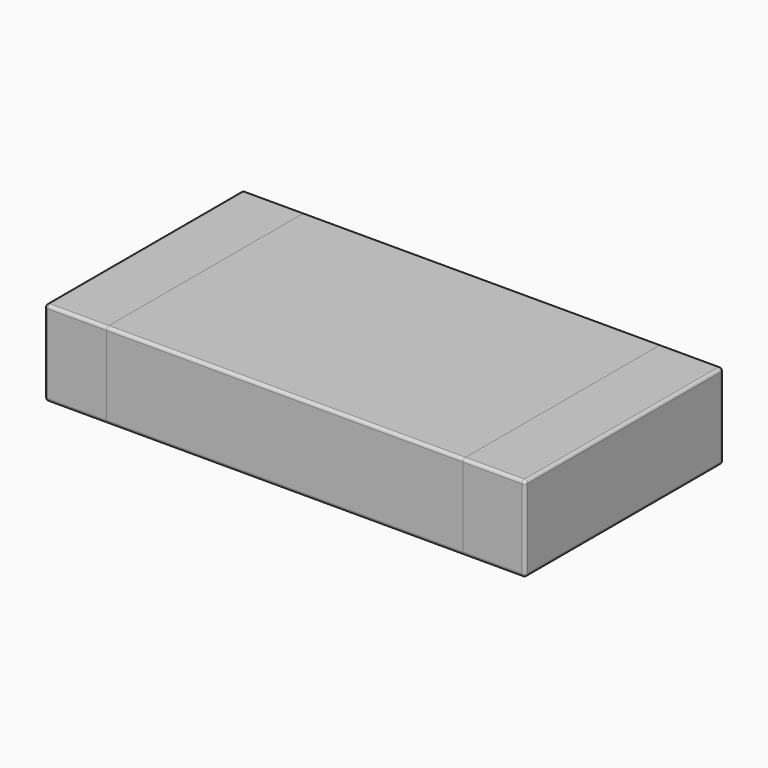
from build123d import *

# Parameters (mm, degrees)
F2_W     = 2.3
F2_H     = 1.6
F3_DEPTH = 0.53
F2_W_2   = 0.4
F4_DEPTH = 0.55
F5_DEPTH = 0.55
F6_DEPTH = 0.02
F7_R     = 0.01999
F7_2_R   = 0.01999
F7_3_R   = 0.01999
F7_4_R   = 0.01999


# Not quite as in the source:
# - a fillet or chamfer is up to 0.001 mm smaller than in the source, because OpenCascade refuses the exact size


with BuildPart() as f3:
    # F2 (on Top) → F3 (new body)
    with BuildSketch(Plane.XY):
        Rectangle(F2_W, F2_H)
    extrude(amount=F3_DEPTH)


with BuildPart() as f4:
    # F2 (on Top) → F4 (new body)
    with BuildSketch(Plane.XY):
        with Locations((-1.35, 0)):
            Rectangle(F2_W_2, F2_H)
    extrude(amount=F4_DEPTH)

    # F7 (radius 0.02 in the source; OpenCascade refuses exactly that, so slightly less here)
    f7_edges = [f4.edges().sort_by_distance(p)[0] for p in [
        (-1.35, -0.8, 0.55),
        (-1.55, 0.8, 0.275),
        (-1.55, -0.8, 0.275),
        (-1.55, 0, 0),
        (-1.55, 0, 0.55),
        (-1.35, 0.8, 0.55),
        (-1.35, 0.8, 0),
        (-1.35, -0.8, 0),
    ]]
    fillet(f7_edges, radius=F7_R)


with BuildPart() as f5:
    # F2 (on Top) → F5 (new body)
    with BuildSketch(Plane.XY):
        with Locations((1.35, 0)):
            Rectangle(F2_W_2, F2_H)
    extrude(amount=F5_DEPTH)

    # F7#2 (radius 0.02 in the source; OpenCascade refuses exactly that, so slightly less here)
    f7_2_edges = [f5.edges().sort_by_distance(p)[0] for p in [
        (1.35, -0.8, 0.55),
        (1.55, -0.8, 0.275),
        (1.55, 0.8, 0.275),
        (1.55, 0, 0),
        (1.55, 0, 0.55),
        (1.35, 0.8, 0.55),
        (1.35, 0.8, 0),
        (1.35, -0.8, 0),
    ]]
    fillet(f7_2_edges, radius=F7_2_R)


with BuildPart() as f6:
    # F6 (new): a face of the model
    f6_faces = [f3.part.faces().sort_by_distance(p)[0] for p in [
        (0, 0, 0.53),
    ]]
    extrude(f6_faces, amount=F6_DEPTH)

    # F7#4 (radius 0.02 in the source; OpenCascade refuses exactly that, so slightly less here)
    f7_4_edges = [f6.edges().sort_by_distance(p)[0] for p in [
        (0, -0.8, 0.55),
        (0, 0.8, 0.55),
    ]]
    fillet(f7_4_edges, radius=F7_4_R)


with BuildPart() as f3_1:
    add(f3.part)

    # F7#3 (radius 0.02 in the source; OpenCascade refuses exactly that, so slightly less here)
    f7_3_edges = [f3_1.edges().sort_by_distance(p)[0] for p in [
        (0, 0.8, 0),
        (0, -0.8, 0),
    ]]
    fillet(f7_3_edges, radius=F7_3_R)


solid = Compound([f4.part, f5.part, f6.part, f3_1.part])
